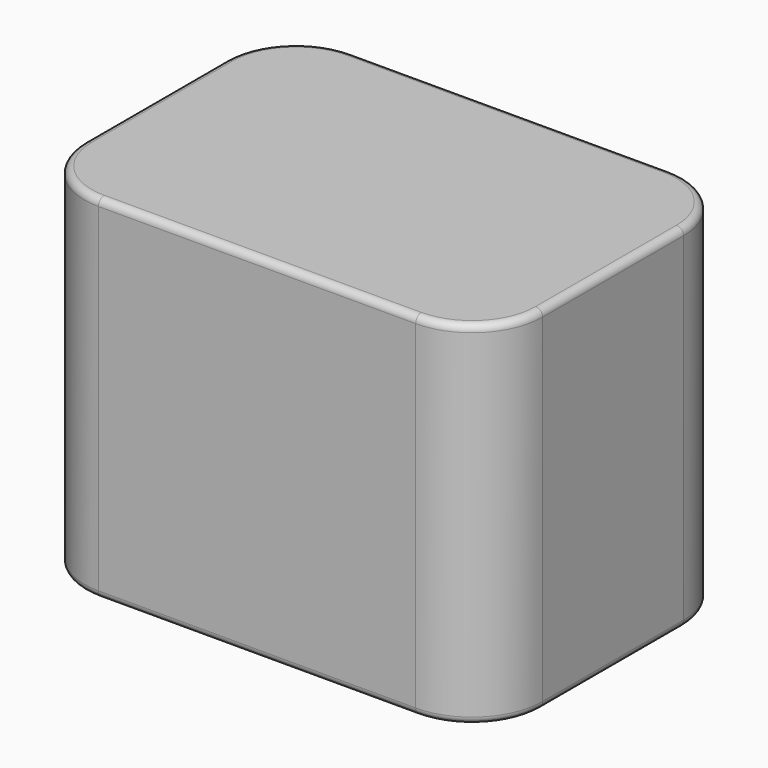
from build123d import *

# Parameters (mm, degrees)
F0_W     = 65
F0_H     = 45
F1_DEPTH = 50
F2_R     = 10
F3_T     = -5
F4_W     = 50
F4_H     = 1.5
F5_DEPTH = 5
F6_R     = 1
F7_F1_R  = 0.7499
F7_F2_R  = 0.75
F8_R     = 2


# Not quite as in the source:
# - a fillet or chamfer is up to 0.001 mm smaller than in the source, because OpenCascade refuses the exact size


with BuildPart() as f1:
    # F0 (on Top) → F1 (new body)
    with BuildSketch(Plane.XY):
        Rectangle(F0_W, F0_H)
    extrude(amount=F1_DEPTH)

    # F2
    f2_edges = [f1.edges().sort_by_distance(p)[0] for p in [
        (32.5, -22.5, 25),
        (-32.5, -22.5, 25),
        (-32.5, 22.5, 25),
        (32.5, 22.5, 25),
    ]]
    fillet(f2_edges, radius=F2_R)

    # F3 (hollow: no face is removed)
    offset(amount=F3_T, mode=Mode.SUBTRACT)

    # F4 (on face) → F5 (cut, through all)
    with BuildSketch(Plane(origin=(0, 0, 0), x_dir=(1, 0, 0), z_dir=(0, 0, -1))):
        with Locations((0, -2.25)):
            Rectangle(F4_W, F4_H)
    extrude(amount=-F5_DEPTH, mode=Mode.SUBTRACT)

    # F6
    f6_edges = [f1.edges().sort_by_distance(p)[0] for p in [
        (0, -22.5, 0),
        (32.5, 0, 50),
        (29.571068, -19.571068, 50),
        (29.571068, 19.571068, 50),
        (0, -22.5, 50),
        (0, 22.5, 50),
        (-29.571068, -19.571068, 50),
        (-29.571068, 19.571068, 50),
        (-32.5, 0, 50),
        (32.5, 0, 0),
        (29.571068, -19.571068, 0),
        (29.571068, 19.571068, 0),
        (0, 22.5, 0),
        (-29.571068, -19.571068, 0),
        (-29.571068, 19.571068, 0),
        (-32.5, 0, 0),
    ]]
    fillet(f6_edges, radius=F6_R)

    # F7: fillet of radius 0.75 on 6 edges, made by hand

    # F7_f1 (radius 0.75 in the source; OpenCascade refuses exactly that, so slightly less here)
    f7_f1_edges = [f1.edges().sort_by_distance(p)[0] for p in [
        (-25, 1.5, 2.5),
        (-25, 3, 2.5),
        (25, 3, 2.5),
        (25, 1.5, 2.5),
    ]]
    fillet(f7_f1_edges, radius=F7_F1_R)

    # F7_f2
    f7_f2_edges = [f1.edges().sort_by_distance(p)[0] for p in [
        (0, 1.5, 0),
        (0, 3, 0),
        (-24.7803593752, 2.7803593752, 0),
        (24.7803593752, 2.7803593752, 0),
        (24.7803593752, 1.7196406248, 0),
        (-24.7803593752, 1.7196406248, 0),
    ]]
    fillet(f7_f2_edges, radius=F7_F2_R)

    # F8
    f8_edges = [f1.edges().sort_by_distance(p)[0] for p in [
        (27.5, 0, 5),
        (0, 17.5, 45),
        (26.035534, 16.035534, 5),
        (26.035534, -16.035534, 5),
        (0, 17.5, 5),
        (0, -17.5, 5),
        (-26.035534, 16.035534, 5),
        (-26.035534, -16.035534, 5),
        (-27.5, 0, 5),
        (27.5, 0, 45),
        (26.035534, 16.035534, 45),
        (26.035534, -16.035534, 45),
        (0, -17.5, 45),
        (-26.035534, 16.035534, 45),
        (-26.035534, -16.035534, 45),
        (-27.5, 0, 45),
    ]]
    fillet(f8_edges, radius=F8_R)


solid = f1.part
